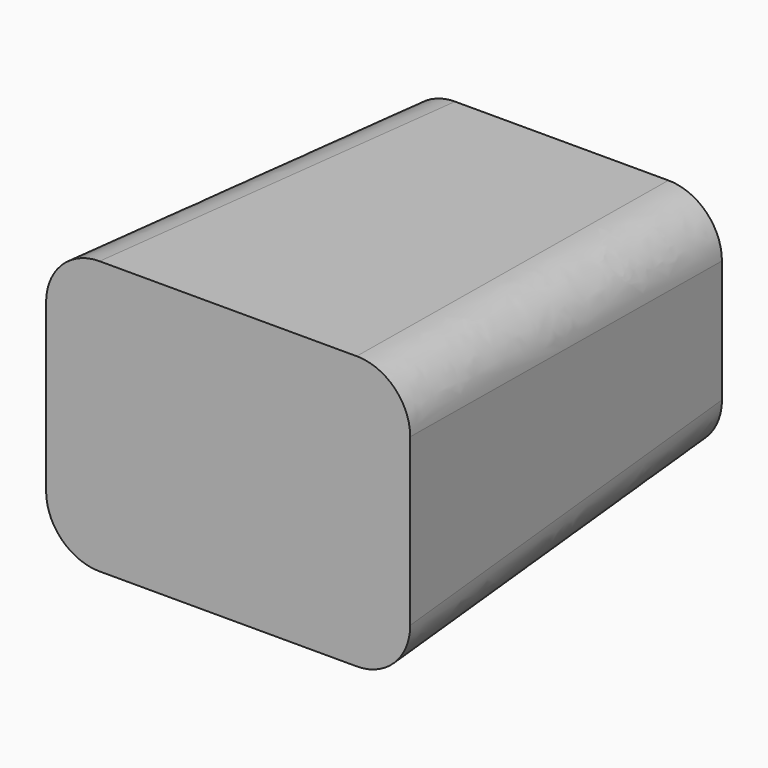
from build123d import *

# Parameters (mm, degrees)
F0_W     = 75.9293138981
F0_H     = 54.3537810445
F1_DEPTH = 98.8087579608
F1_TAPER = -3
F2_R     = 12.7


with BuildPart() as f1:
    # F0 (on Front) → F1 (new body)
    with BuildSketch(Plane.XZ):
        with Locations((-0.829860568, 9.5430351794)):
            Rectangle(F0_W, F0_H)
    extrude(amount=F1_DEPTH, taper=F1_TAPER)

    # F2
    f2_edges = [f1.edges().sort_by_distance(p)[0] for p in [
        (39.72397, -49.404379, 39.309099),
        (-41.383691, -49.404379, 39.309099),
        (39.72397, -49.404379, -20.223029),
        (-41.383691, -49.404379, -20.223029),
    ]]
    fillet(f2_edges, radius=F2_R)


solid = f1.part
